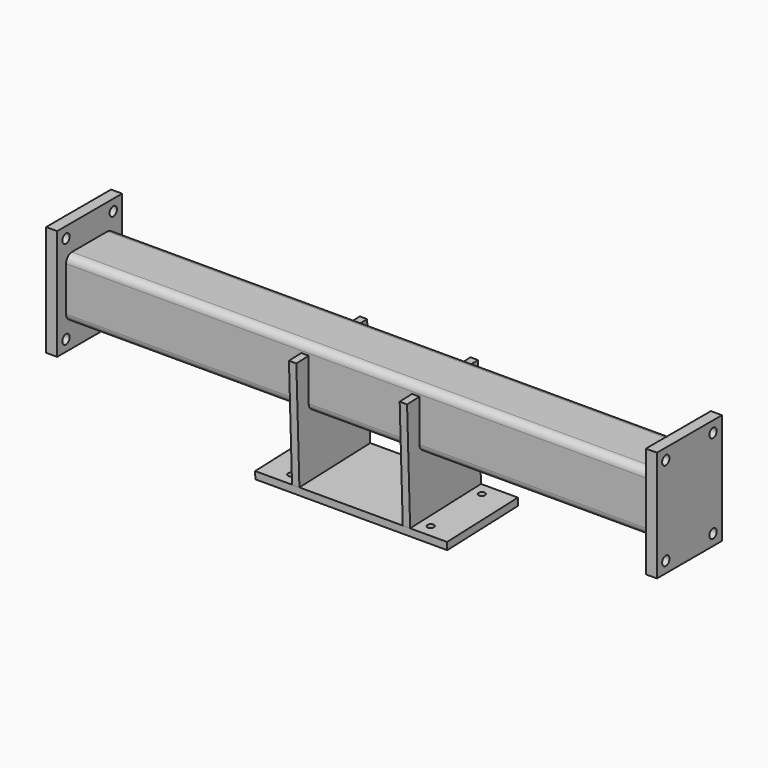
from build123d import *

# Parameters (mm, degrees)
F1_DEPTH  = 506.4125
F2_W      = 139.7
F2_H      = 190.5
F3_DEPTH  = 19.05
F5_D      = 15.875
F9_DEPTH  = 12.7
F11_W     = 330.2
F11_H     = 152.4
F12_DEPTH = 12.7
F14_D     = 11.1125


# Not quite as in the source:
# - a length typed as a fraction of an inch, garbled in the dataset ("3 / 203.2 mm" for 3/8 in), is restored


with BuildPart() as f1:
    # F0 (on Right) → F1 (new body, symmetric)
    with BuildSketch(Plane.YZ):
        with BuildLine():
            Line((38.1, 50.8), (-38.1, 50.8))
            ThreePointArc((-38.1, 50.8), (-47.0802561211, 47.0802561211), (-50.8, 38.1))
            Line((-50.8, 38.1), (-50.8, -38.1))
            ThreePointArc((-50.8, -38.1), (-47.0802561211, -47.0802561211), (-38.1, -50.8))
            Line((-38.1, -50.8), (38.1, -50.8))
            ThreePointArc((38.1, -50.8), (47.0802561211, -47.0802561211), (50.8, -38.1))
            Line((50.8, -38.1), (50.8, 38.1))
            ThreePointArc((50.8, 38.1), (47.0802561211, 47.0802561211), (38.1, 50.8))
        make_face()
        with BuildLine():
            ThreePointArc((-44.45, 38.1), (-42.5901280605, 42.5901280605), (-38.1, 44.45))
            Line((-38.1, 44.45), (38.1, 44.45))
            ThreePointArc((38.1, 44.45), (42.5901280605, 42.5901280605), (44.45, 38.1))
            Line((44.45, 38.1), (44.45, -38.1))
            ThreePointArc((44.45, -38.1), (42.5901280605, -42.5901280605), (38.1, -44.45))
            Line((38.1, -44.45), (-38.1, -44.45))
            ThreePointArc((-38.1, -44.45), (-42.5901280605, -42.5901280605), (-44.45, -38.1))
            Line((-44.45, -38.1), (-44.45, 38.1))
        make_face(mode=Mode.SUBTRACT)
    extrude(amount=F1_DEPTH, both=True)


with BuildPart() as f3:
    # F2 (on face) → F3 (new body)
    with BuildSketch(Plane.YZ.offset(506.4125)):
        Rectangle(F2_W, F2_H)
    extrude(amount=F3_DEPTH)

    # F5 (through all)
    with Locations(Plane.YZ.offset(525.4625)):
        with Locations((-50.8, 76.2), (50.8, 76.2), (-50.8, -76.2), (50.8, -76.2)):
            Hole(F5_D / 2)


with BuildPart() as f6_1:
    # F6: instance of F3
    add(f3.part.mirror(Plane.YZ))


with BuildPart() as f9:
    # F8 (on offset) → F9 (new body)
    with BuildSketch(Plane.YZ.offset(88.9)):
        with BuildLine():
            Line((81.5349474393, -151.4428301741), (74.8865933174, 38.9411223731))
            Line((74.8865933174, 38.9411223731), (50.8, 38.1))
            Line((50.8, 38.1), (50.8, -38.1))
            ThreePointArc((50.8, -38.1), (47.0802561211, -47.0802561211), (38.1, -50.8))
            Line((38.1, -50.8), (-38.1, -50.8))
            ThreePointArc((-38.1, -50.8), (-47.0802561211, -47.0802561211), (-50.8, -38.1))
            Line((-50.8, -38.1), (-50.8, 34.5520498196))
            Line((-50.8, 34.5520498196), (-77.4205687203, 33.6224390756))
            Line((-77.4205687203, 33.6224390756), (-70.7722145985, -156.7615134715))
            Line((-70.7722145985, -156.7615134715), (81.5349474393, -151.4428301741))
        make_face()
    extrude(amount=F9_DEPTH)


with BuildPart() as f10_1:
    # F10: instance of F9
    add(f9.part.mirror(Plane.YZ))


with BuildPart() as f12:
    # F11 (on face) → F12 (new body)
    with BuildSketch(Plane(origin=(0, 5.3813664204, -154.1021718228), x_dir=(1, 0, 0), z_dir=(0, 0.0348994967, -0.999390827))):
        Rectangle(F11_W, F11_H)
    extrude(amount=F12_DEPTH)

    # F14 (through all)
    with Locations(Plane(origin=(0, 5.8245900285, -166.7944353259), x_dir=(1, 0, 0), z_dir=(0, 0.0348994967, -0.999390827))):
        with Locations((-120.015, 54.991), (120.015, 54.991), (120.015, -54.991), (-120.015, -54.991)):
            Hole(F14_D / 2)


solid = Compound([f1.part, f3.part, f6_1.part, f9.part, f10_1.part, f12.part])
